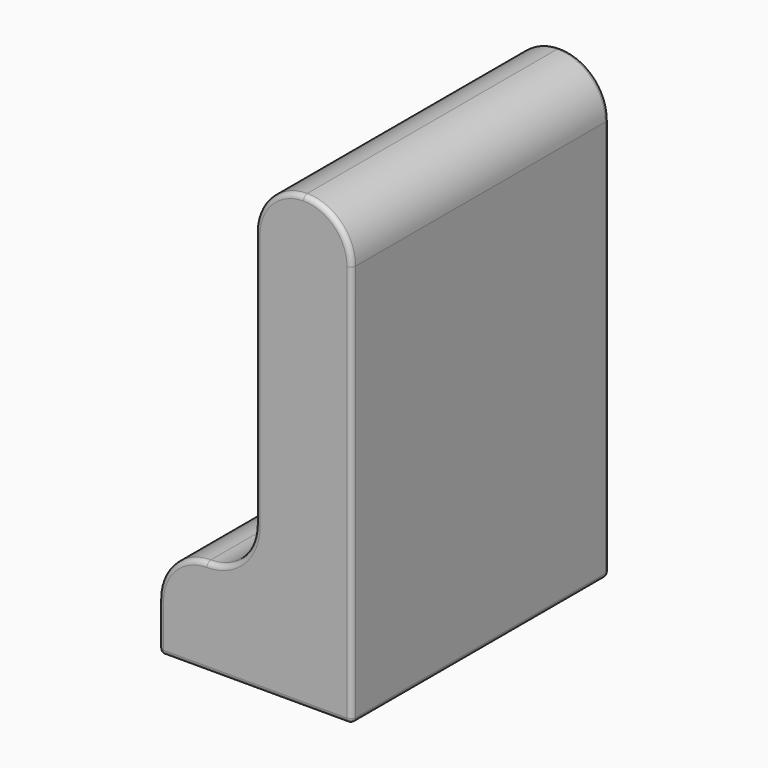
from build123d import *

# Parameters (mm, degrees)
F0_W     = 30
F0_H     = 110
F1_DEPTH = 100
F2_R     = 14.99999
F3_R     = 14.99999
F4_R     = 1.5


# Not quite as in the source:
# - a fillet or chamfer is up to 0.001 mm smaller than in the source, because OpenCascade refuses the exact size


with BuildPart() as f1:
    # F0 (on Front) → F1 (new body)
    with BuildSketch(Plane.XZ):
        Polygon((-60, 0), (0, 0), (0, 30), (-30, 30), (-60, 30), align=None)
        with Locations((-15, 85)):
            Rectangle(F0_W, F0_H)
    extrude(amount=F1_DEPTH)

    # F2 (radius 15 in the source; OpenCascade refuses exactly that, so slightly less here)
    f2_edges = [f1.edges().sort_by_distance(p)[0] for p in [
        (-30, -50, 30),
        (-60, -50, 30),
    ]]
    fillet(f2_edges, radius=F2_R)

    # F3 (radius 15 in the source; OpenCascade refuses exactly that, so slightly less here)
    f3_edges = [f1.edges().sort_by_distance(p)[0] for p in [
        (-30, -50, 140),
        (0, -50, 140),
    ]]
    fillet(f3_edges, radius=F3_R)

    # F4
    f4_edges = [f1.edges().sort_by_distance(p)[0] for p in [
        (0, -50, 0),
        (-30, -100, 0),
        (-60, -50, 0),
        (-30, 0, 0),
        (0, -100, 62.500005),
        (0, 0, 62.500005),
    ]]
    fillet(f4_edges, radius=F4_R)


solid = f1.part
